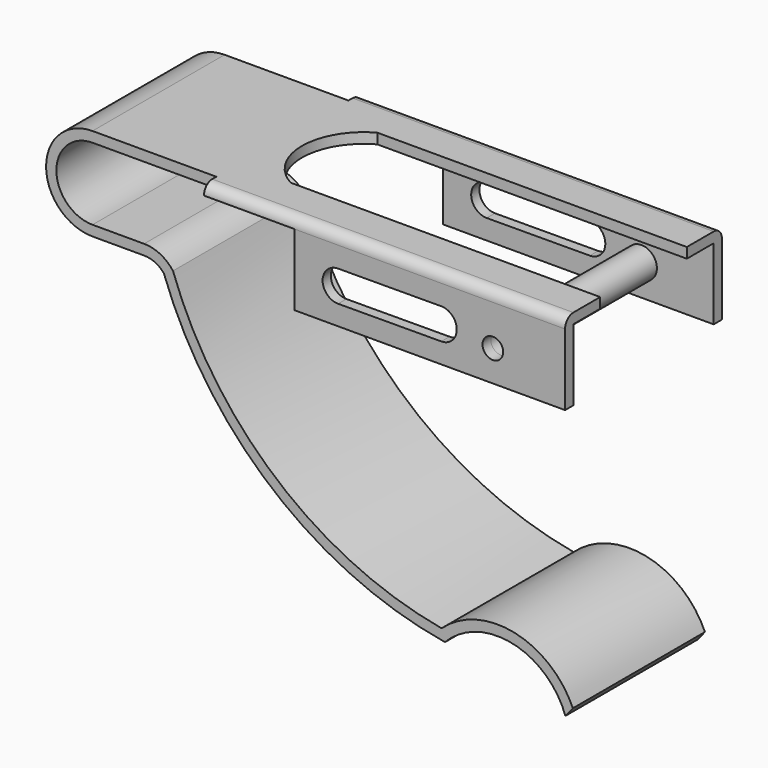
from build123d import *

# Parameters (mm, degrees)
F1_DEPTH  = 16
F2_W      = 70
F2_H      = 3
F3_DEPTH  = 2
F4_W      = 52.4458656609
F4_H      = 13.8459985778
F5_DEPTH  = 2
F8_DEPTH  = 2
F9_R      = 2
F11_DEPTH = 38.001
F13_D     = 4
F14_R     = 3
F14_R_2   = 2
F15_DEPTH = 34.5


with BuildPart() as f1:
    # F0 (on Front) → F1 (new body)
    with BuildSketch(Plane.XZ):
        with BuildLine():
            Line((94, 9), (0, 9))
            ThreePointArc((0, 9), (-9, 0), (0, -9))
            Line((0, -9), (10, -9))
            ThreePointArc((10, -9), (12.1096761181, -9.4668701015), (13.8253743549, -10.7802933293))
            ThreePointArc((13.8253743549, -10.7802933293), (34.9359413113, -40.7908803671), (68.327168476, -56))
            ThreePointArc((68.327168476, -56), (81.3946239912, -51.9695299334), (91.6636888451, -61))
            Line((91.6636888451, -61), (93.1092569516, -59.2209782))
            ThreePointArc((93.1092569516, -59.2209782), (81.7616044026, -50.0028575081), (67.6586675506, -53.8564453964))
            ThreePointArc((67.6586675506, -53.8564453964), (35.7039452814, -38.8251123565), (15.5964314226, -9.7952461033))
            ThreePointArc((15.5964314226, -9.7952461033), (13.1278365305, -7.7376810494), (10, -7))
            Line((10, -7), (0, -7))
            ThreePointArc((0, -7), (-7, 0), (0, 7))
            Line((0, 7), (94, 7))
            Line((94, 7), (94, 9))
        make_face()
    extrude(amount=F1_DEPTH)

    # F2 (on face) → F3 (join)
    with BuildSketch(Plane.XY.offset(9)):
        with Locations((59, -17.5)):
            Rectangle(F2_W, F2_H)
    extrude(amount=-F3_DEPTH)

    # F4 (on face) → F5 (join)
    with BuildSketch(Plane.XZ.offset(19)):
        with Locations((67.7770671695, 0.0770007111)):
            Rectangle(F4_W, F4_H)
    extrude(amount=-F5_DEPTH)

    # F6: F1 across face


with BuildPart() as f1_1:
    add(f1.part)
    add(f1.part.mirror(Plane(origin=(40.1817011291, 0, -15.4832521129), x_dir=(1, 0, 0), z_dir=(0, 1, 0))))

    # F7 (on face) → F8 (cut)
    with BuildSketch(Plane.XY.offset(9)):
        with BuildLine():
            Line((34, -10.5), (94, -10.5))
            Line((94, -10.5), (94, 10.5))
            Line((94, 10.5), (34, 10.5))
            ThreePointArc((34, 10.5), (27.8094750193, 0), (34, -10.5))
        make_face()
    extrude(amount=-F8_DEPTH, mode=Mode.SUBTRACT)

    # F9
    f9_edges = [f1_1.edges().sort_by_distance(p)[0] for p in [
        (59, -19, 9),
        (59, 19, 9),
    ]]
    fillet(f9_edges, radius=F9_R)

    # F10 (on face) → F11 (cut, through all)
    with BuildSketch(Plane.XZ.offset(19)):
        with BuildLine():
            ThreePointArc((70.0115500211, -2.922977055), (72.9999777661, 0.0885507322), (69.9884499789, 3.0769784772))
            Line((69.9884499789, 3.0769784772), (49.9884499789, 2.9999777661))
            ThreePointArc((49.9884499789, 2.9999777661), (47.0000222339, -0.0115500211), (50.0115500211, -2.9999777661))
            Line((50.0115500211, -2.9999777661), (70.0115500211, -2.922977055))
        make_face()
    extrude(amount=-F11_DEPTH, mode=Mode.SUBTRACT)

    # F13 (through all)
    with Locations(Plane(origin=(0, 19, 0), x_dir=(-1, 0, 0), z_dir=(0, 1, 0))):
        with Locations((-80, -0.8459985778)):
            Hole(F13_D / 2)

    # F14 (on face) → F15 (join)
    with BuildSketch(Plane(origin=(0, -17, 0), x_dir=(-1, 0, 0), z_dir=(0, 1, 0))):
        with Locations((-80, -0.8459985778)):
            Circle(F14_R)
        with Locations((-80, -0.8459985778)):
            Circle(F14_R_2, mode=Mode.SUBTRACT)
    extrude(amount=F15_DEPTH)


solid = f1_1.part
